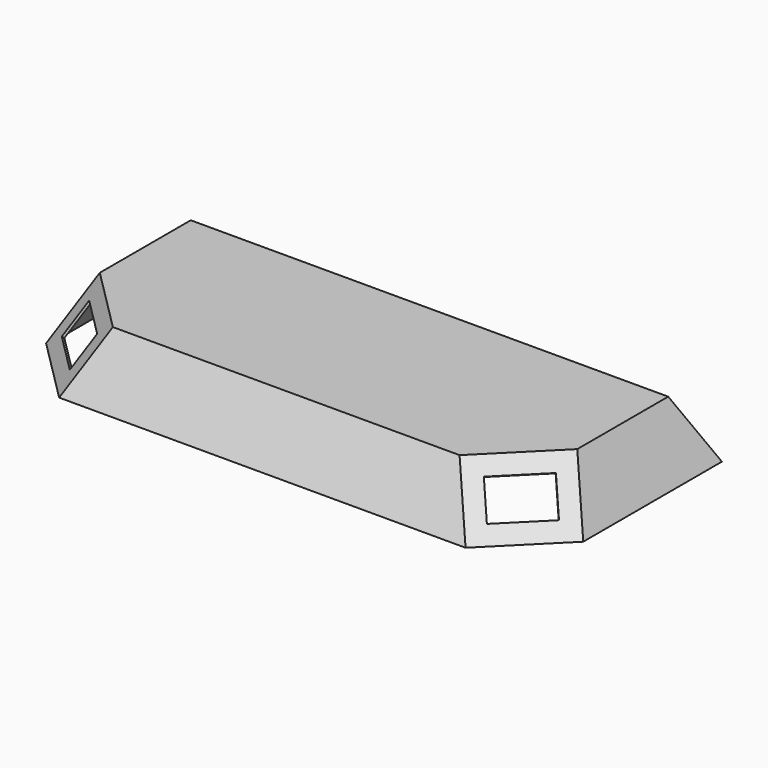
from build123d import *

# Parameters (mm, degrees)
F0_W     = 2743.2
F0_H     = 1219.2
F2_W     = 2438.4
F2_H     = 914.4
F4_SIZE  = 304.8
F5_T     = -12.7
F8_DEPTH = 2120.3111006463


# Not quite as in the source:
# - a pattern or mirror of a feature is missing from the dataset's text; its kind, count and spacing are read off the source's solid


with BuildPart() as f3:
    # F0 (on Top) → F3 section 0
    with BuildSketch(Plane.XY):
        Rectangle(F0_W, F0_H)
    # F2 (on offset) → F3 section 1
    with BuildSketch(Plane.XY.offset(304.8)):
        Rectangle(F2_W, F2_H)
    loft()

    # F4
    f4_edges = [f3.edges().sort_by_distance(p)[0] for p in [
        (1295.4, -533.4, 152.4),
        (-1295.4, -533.4, 152.4),
    ]]
    chamfer(f4_edges, length=F4_SIZE)

    # F5
    f5_openings = [f3.faces().sort_by_distance(p)[0] for p in [
        (0, 17.182854, 0),
    ]]
    offset(amount=F5_T, openings=f5_openings, kind=Kind.INTERSECTION)

    # F7 (on face) → F8 (cut, through all)
    with BuildSketch(Plane(origin=(-563.7616072736, -563.7616072736, 563.7616072736), x_dir=(0.8164965809, -0.4082482905, 0.4082482905), z_dir=(-0.5773502692, -0.5773502692, 0.5773502692))):
        Polygon((-536.6753892389, -141.2324363749), (-787.22877512, 3.4246284099), (-882.43989352, -161.4858661045), (-631.886507639, -306.1429308893), align=None)
    f8 = extrude(amount=-F8_DEPTH, mode=Mode.SUBTRACT)

    # F8_copies: F8 across plane
    add(f8.mirror(Plane(origin=(0, 0, 0), x_dir=(0, 0, 1), z_dir=(1, 0, 0))), mode=Mode.SUBTRACT)


solid = f3.part
